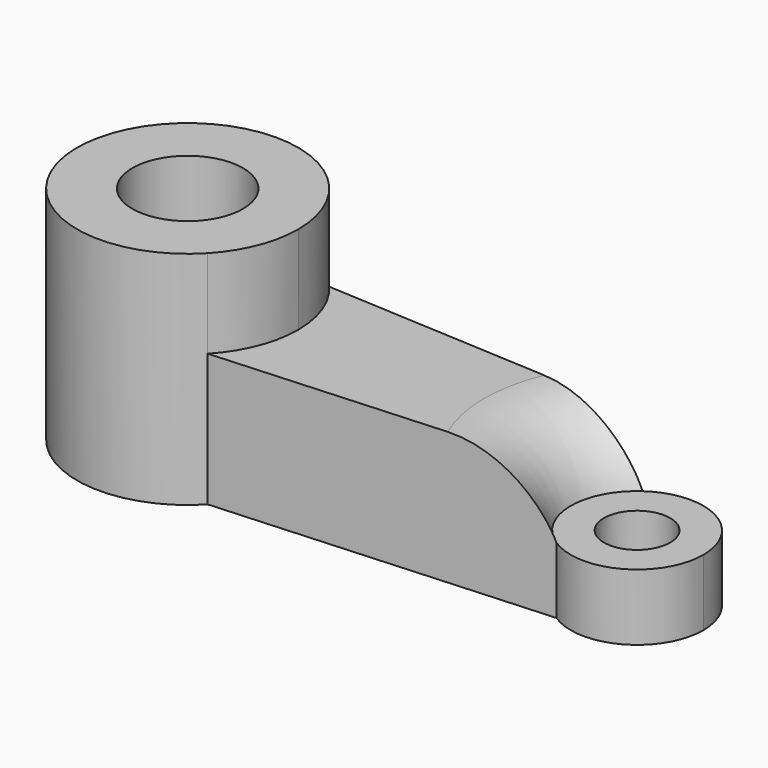
from build123d import *

# Parameters (mm, degrees)
F0_R        = 6.25
F1_DEPTH    = 25
F2_DEPTH    = 15
F0_R_2      = 3.75
F3_DEPTH    = 7.5
F4_T2_ANGLE = 359.64


# Not quite as in the source:
# - a fillet or chamfer that OpenCascade refuses, or shapes differently, is made with other operations: its cross-section is extruded or revolved along the edge and cut away or added


with BuildPart() as f1:
    # F0 (on Top) → F1 (new body)
    with BuildSketch(Plane.XY):
        with BuildLine():
            ThreePointArc((-20.8125196211, -8.5595397618), (-18.3005664883, -4.6032795782), (-17.4220903611, 0))
            ThreePointArc((-17.4220903611, 0), (-18.1998915609, 4.3405132519), (-20.4364992075, 8.1408574773))
            ThreePointArc((-20.4364992075, 8.1408574773), (-42.4189230977, 0.2813743978), (-20.8125196211, -8.5595397618))
        make_face()
        with Locations((-29.9220903611, 0)):
            Circle(F0_R, mode=Mode.SUBTRACT)
    extrude(amount=F1_DEPTH)

    # F0 (on Top) → F2 (join)
    with BuildSketch(Plane.XY):
        with BuildLine():
            ThreePointArc((-20.4364992075, 8.1408574773), (-18.1998915609, 4.3405132519), (-17.4220903611, 0))
            ThreePointArc((-17.4220903611, 0), (-18.3005664883, -4.6032795782), (-20.8125196211, -8.5595397618))
            Line((-20.8125196211, -8.5595397618), (16.7775256305, -6.2798766695))
            ThreePointArc((16.7775256305, -6.2798766695), (13.3788672096, -0.1198442426), (16.5789499879, 6.1456444673))
            Line((16.5789499879, 6.1456444673), (-20.4364992075, 8.1408574773))
        make_face()
    extrude(amount=F2_DEPTH)

    # F0 (on Top) → F3 (join)
    with BuildSketch(Plane.XY):
        with BuildLine():
            ThreePointArc((28.3779096389, 0), (24.3425743137, 6.651774101), (16.5789499879, 6.1456444673))
            ThreePointArc((16.5789499879, 6.1456444673), (13.3788672096, -0.1198442426), (16.7775256305, -6.2798766695))
            ThreePointArc((16.7775256305, -6.2798766695), (24.4484222028, -6.5955621467), (28.3779096389, 0))
        make_face()
        with Locations((20.8779096389, 0)):
            Circle(F0_R_2, mode=Mode.SUBTRACT)
    extrude(amount=F3_DEPTH)

    # F4: fillet of radius 10.139696962 on 1 edges, made by hand

    # F4_s1 → F4_t2 (revolve, cut)
    with BuildSketch(Plane(origin=(0.0034409593, -0.268007829, 0), x_dir=(0, 0, 1), z_dir=(-0.0128379671, 0.9999175899, 0))):
        with BuildLine():
            ThreePointArc((15, 38.1662582623), (12.909501189, 31.999908969), (7.5, 28.3761890884))
            Line((7.5, 28.3761890884), (15, 28.3761890884))
            Line((15, 28.3761890884), (15, 38.1662582623))
        make_face()
    revolve(axis=Axis((20.8779096389, 0, 15), (0, 0, -1)), revolution_arc=F4_T2_ANGLE, mode=Mode.SUBTRACT)


solid = f1.part
